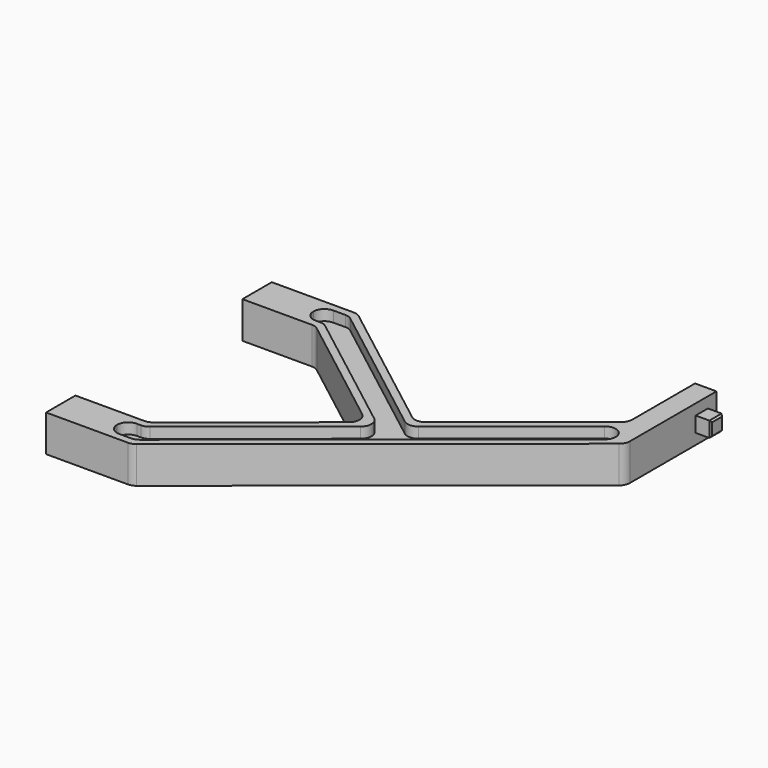
from build123d import *

# Parameters (mm, degrees)
F1_DEPTH = 3.81
F2_DEPTH = 1.5875
F0_W     = 3.175
F0_H     = 3.175
F3_DEPTH = 1.5875
F4_R     = 2.28599
F5_SIZE  = 0.3302


# Not quite as in the source:
# - a fillet or chamfer is up to 0.001 mm smaller than in the source, because OpenCascade refuses the exact size


with BuildPart() as f1:
    # F0 (on Top) → F1 (new body, symmetric)
    with BuildSketch(Plane.XY):
        Polygon((0, 17.9811139863), (0, 10.3611139863), (17.78, 10.3611139863), (80.1876843047, 60.4647179591), (80.1876843047, 78.6070511723), (80.1876843047, 81.7820511723), (80.1876843047, 84.0045511723), (75.7426843047, 84.0045511723), (75.7426843047, 66.6679901496), (48.789068088, 45.0284544481), (17.78, 68.9081139863), (0, 68.9081139863), (0, 61.2881139863), (15.1859866786, 61.2881139863), (15.5029622538, 61.0440154278), (42.6746095935, 40.1195011625), (17.78, 20.1330255541), (15.0996375684, 17.9811139863), align=None)
        Polygon((11.684, 67.3841139863), (17.2611973357, 67.3841139863), (48.8086871908, 43.0898232038), (75.5083847301, 64.5255019445), (78.3706676759, 60.9603202747), (17.2439275137, 11.8851139863), (11.684, 11.8851139863), (11.684, 16.4571139863), (15.6357100547, 16.4571139863), (45.1400120941, 40.1444512324), (15.7047893428, 62.8121139863), (11.684, 62.8121139863), align=None, mode=Mode.SUBTRACT)
    extrude(amount=F1_DEPTH, both=True)

    # F0 (on Top) → F2 (join, symmetric)
    with BuildSketch(Plane.XY):
        Polygon((48.8086871908, 43.0898232038), (17.2611973357, 67.3841139863), (11.684, 67.3841139863), (11.684, 62.8121139863), (15.7047893428, 62.8121139863), (45.1400120941, 40.1444512324), (15.6357100547, 16.4571139863), (11.684, 16.4571139863), (11.684, 11.8851139863), (17.2439275137, 11.8851139863), (78.3706676759, 60.9603202747), (75.5083847301, 64.5255019445), align=None)
    extrude(amount=F2_DEPTH, both=True)

    # F0 (on Top) → F3 (join, symmetric)
    with BuildSketch(Plane.XY):
        with Locations((81.7751843047, 80.1945511723)):
            Rectangle(F0_W, F0_H)
    extrude(amount=F3_DEPTH, both=True)

    # F4 (radius 2.286 in the source; OpenCascade refuses exactly that, so slightly less here)
    f4_edges = [f1.edges().sort_by_distance(p)[0] for p in [
        (15.185987, 61.288114, 0),
        (11.684, 62.812114, 2.69875),
        (15.704789, 62.812114, 2.69875),
        (11.684, 67.384114, 2.69875),
        (17.261197, 67.384114, 2.69875),
        (17.78, 68.908114, 0),
        (15.704789, 62.812114, -2.69875),
        (11.684, 62.812114, -2.69875),
        (11.684, 67.384114, -2.69875),
        (17.261197, 67.384114, -2.69875),
        (48.808687, 43.089823, 2.69875),
        (45.140012, 40.144451, 2.69875),
        (42.67461, 40.119501, 0),
        (48.789068, 45.028454, 0),
        (48.808687, 43.089823, -2.69875),
        (45.140012, 40.144451, -2.69875),
        (75.508385, 64.525502, -2.69875),
        (78.370668, 60.96032, -2.69875),
        (80.187684, 60.464718, 0),
        (75.742684, 66.66799, 0),
        (78.370668, 60.96032, 2.69875),
        (75.508385, 64.525502, 2.69875),
        (15.63571, 16.457114, 2.69875),
        (11.684, 16.457114, 2.69875),
        (11.684, 11.885114, 2.69875),
        (17.243928, 11.885114, 2.69875),
        (11.684, 16.457114, -2.69875),
        (15.63571, 16.457114, -2.69875),
        (17.243928, 11.885114, -2.69875),
        (11.684, 11.885114, -2.69875),
        (17.78, 10.361114, 0),
        (15.099638, 17.981114, 0),
    ]]
    fillet(f4_edges, radius=F4_R)

    # F5
    f5_edges = [f1.edges().sort_by_distance(p)[0] for p in [
        (83.362684, 78.607051, 0),
        (83.362684, 80.194551, -1.5875),
        (83.362684, 81.782051, 0),
        (83.362684, 80.194551, 1.5875),
    ]]
    chamfer(f5_edges, length=F5_SIZE)


with BuildPart() as f1_1:
    # F6: moved
    add(f1.part.moved(Location((0, 0, 3.81))))


solid = f1_1.part
